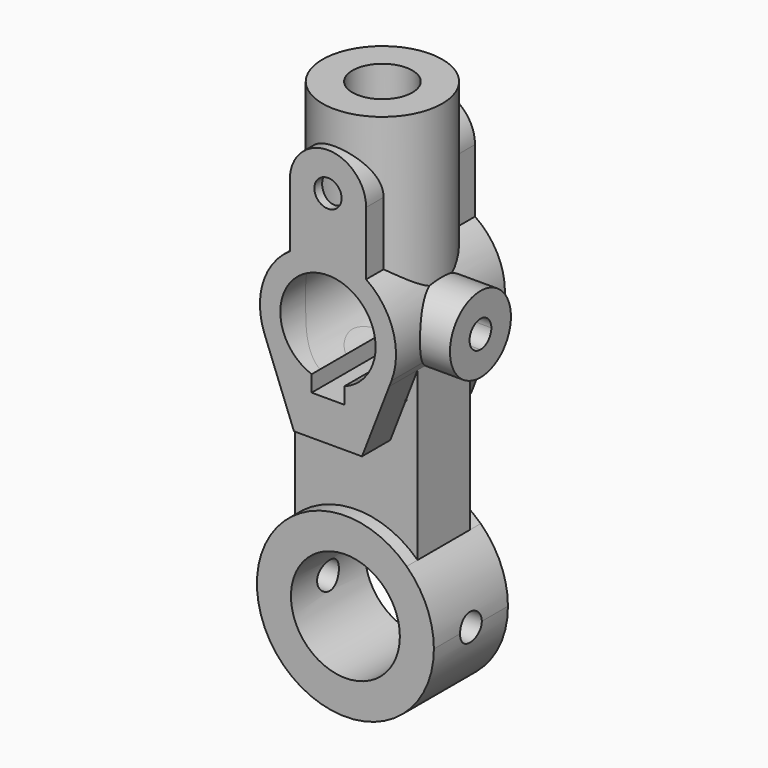
from build123d import *

# Parameters (mm, degrees)
F0_R      = 20
F1_DEPTH  = 17
F2_DEPTH  = 12
F0_R_2    = 5
F3_DEPTH  = 25
F4_R      = 22
F4_R_2    = 11
F5_DEPTH  = 92.4
F8_DEPTH  = 36
F9_DEPTH  = 50.001
F10_R     = 5
F11_DEPTH = 36
F12_R     = 5
F13_DEPTH = 50
F14_R     = 11
F15_DEPTH = 60


with BuildPart() as f1:
    # F0 (on Front) → F1 (new body, symmetric)
    with BuildSketch(Plane.XZ):
        with BuildLine():
            ThreePointArc((-22.5, 23.452079), (-12.747549, -29.895652), (32.5, 0))
            ThreePointArc((32.5, 0), (29.895652, 12.747549), (22.5, 23.452079))
            ThreePointArc((22.5, 23.452079), (0, 32.5), (-22.5, 23.452079))
        make_face()
        Circle(F0_R, mode=Mode.SUBTRACT)
    extrude(amount=F1_DEPTH, both=True)

    # F0 (on Front) → F2 (join, symmetric)
    with BuildSketch(Plane.XZ):
        with BuildLine():
            ThreePointArc((-22.5, 23.452079), (0, 32.5), (22.5, 23.452079))
            Line((22.5, 23.452079), (22.5, 84.869144))
            Line((22.5, 84.869144), (12.5, 59.003379))
            Line((12.5, 59.003379), (-12.5, 59.003379))
            Line((-12.5, 59.003379), (-22.5, 84.869144))
            Line((-22.5, 84.869144), (-22.5, 23.452079))
        make_face()
    extrude(amount=F2_DEPTH, both=True)

    # F0 (on Front) → F3 (join, symmetric)
    with BuildSketch(Plane.XZ):
        with BuildLine():
            Line((12.5, 59.003379), (22.5, 84.869144))
            Line((22.5, 84.869144), (23.318011, 86.984991))
            ThreePointArc((23.318011, 86.984991), (23.855543, 103.477505), (14, 116.712315))
            Line((14, 116.712315), (14, 140))
            ThreePointArc((14, 140), (0, 154), (-14, 140))
            Line((-14, 140), (-14, 116.712315))
            ThreePointArc((-14, 116.712315), (-23.855543, 103.477505), (-23.318011, 86.984991))
            Line((-23.318011, 86.984991), (-22.5, 84.869144))
            Line((-22.5, 84.869144), (-12.5, 59.003379))
            Line((-12.5, 59.003379), (12.5, 59.003379))
        make_face()
        with BuildLine():
            ThreePointArc((-6, 79.560718), (0, 113.5), (6, 79.560718))
            Line((6, 79.560718), (6, 73.6))
            Line((6, 73.6), (-6, 73.6))
            Line((-6, 73.6), (-6, 79.560718))
        make_face(mode=Mode.SUBTRACT)
        with Locations((0, 140)):
            Circle(F0_R_2, mode=Mode.SUBTRACT)
    extrude(amount=F3_DEPTH, both=True)

    # F4 (on face) → F5 (join)
    with BuildSketch(Plane.XY.offset(73.6)):
        Circle(F4_R)
        Circle(F4_R_2, mode=Mode.SUBTRACT)
    extrude(amount=F5_DEPTH)

    # F7 (on Right) → F8 (join)
    with BuildSketch(Plane.YZ):
        with BuildLine():
            ThreePointArc((14, 96), (-9.899495, 105.899495), (0, 82))
            ThreePointArc((0, 82), (9.899495, 86.100505), (14, 96))
        make_face()
        with BuildLine():
            ThreePointArc((5, 96), (3.535534, 92.464466), (0, 91))
            ThreePointArc((0, 91), (-3.535534, 99.535534), (5, 96))
        make_face(mode=Mode.SUBTRACT)
    extrude(amount=F8_DEPTH)

    # F6 (on face) → F9 (cut, through all)
    with BuildSketch(Plane.XZ.offset(25)):
        with BuildLine():
            Line((6, 73.6), (6, 79.560718))
            ThreePointArc((6, 79.560718), (0, 113.5), (-6, 79.560718))
            Line((-6, 79.560718), (-6, 73.6))
            Line((-6, 73.6), (6, 73.6))
        make_face()
    extrude(amount=-F9_DEPTH, mode=Mode.SUBTRACT)

    # F10 (on face) → F11 (cut)
    with BuildSketch(Plane.YZ.offset(36)):
        with Locations((0, 96)):
            Circle(F10_R)
    extrude(amount=-F11_DEPTH, mode=Mode.SUBTRACT)

    # F12 (on Right) → F13 (cut, symmetric)
    with BuildSketch(Plane.YZ):
        Circle(F12_R)
    extrude(amount=F13_DEPTH, both=True, mode=Mode.SUBTRACT)

    # F14 (on face) → F15 (cut)
    with BuildSketch(Plane.XY.offset(166)):
        Circle(F14_R)
    extrude(amount=-F15_DEPTH, mode=Mode.SUBTRACT)


solid = f1.part
